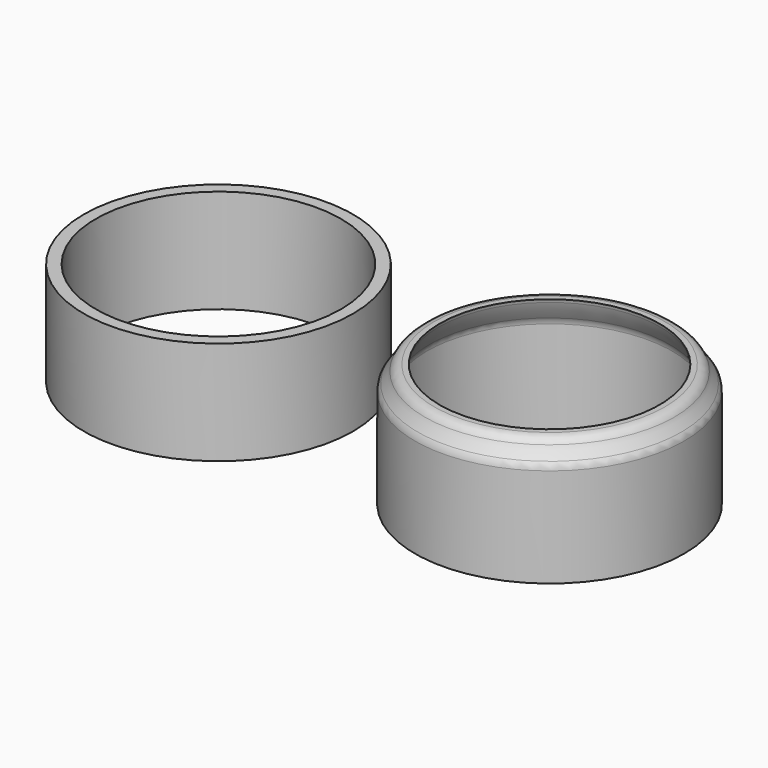
from build123d import *

# Parameters (mm, degrees)
F0_R     = 9.906
F0_R_2   = 9.017
F1_DEPTH = 7.62
F4_R     = 0.762


# Not quite as in the source:
# - ends of sketch curves that miss each other by under 0.0002 mm in the source are joined


with BuildPart() as f1:
    # F0 (on Top) → F1 (new body)
    with BuildSketch(Plane.XY):
        Circle(F0_R)
        Circle(F0_R_2, mode=Mode.SUBTRACT)
    extrude(amount=F1_DEPTH)


with BuildPart() as f3:
    # F2 (on Front) → F3 (revolve)
    with BuildSketch(Plane.XZ):
        with BuildLine():
            Line((14.4612686709, 7.62), (14.4612686709, 0))
            Line((14.4612686709, 0), (15.3502686709, 0))
            Line((15.3502686709, 0), (15.3502686709, 7.2476301639))
            add(Edge.make_bspline(
                [(15.3502686709, 7.2476301639), (15.3919398222, 7.2943099028), (15.563906281, 7.4988239117), (15.8154492473, 7.8746040023), (16.057110979, 8.3604725059), (16.165645556, 8.6639414702), (16.2069450038, 8.812884039)],
                knots=[0.1746961563, 0.1746961563, 0.1746961563, 0.1746961563, 0.25, 0.5, 0.75, 1, 1, 1, 1], degree=3))
            Line((16.2069450038, 8.812884039), (16.274407506, 9.0504270047))
            Line((16.274407506, 9.0504270047), (15.3502686709, 9.0504270047))
            add(Edge.make_bspline(
                [(14.4612686709, 7.62), (14.9159906432, 7.9980511218), (15.2358394116, 8.6377486587), (15.3502686709, 9.0504270047)],
                knots=[0, 0, 0, 0, 1.6841741049, 1.6841741049, 1.6841741049, 1.6841741049], degree=3))
        make_face()
    revolve(axis=Axis((24.3672686709, 0, 3.81), (0, 0, 1)))

    # F4
    f4_edges = [f3.edges().sort_by_distance(p)[0] for p in [
        (34.273269, 0, 7.62),
        (33.384269, 0, 9.050427),
        (33.384269, 0, 7.24763),
    ]]
    fillet(f4_edges, radius=F4_R)


solid = Compound([f1.part, f3.part])
